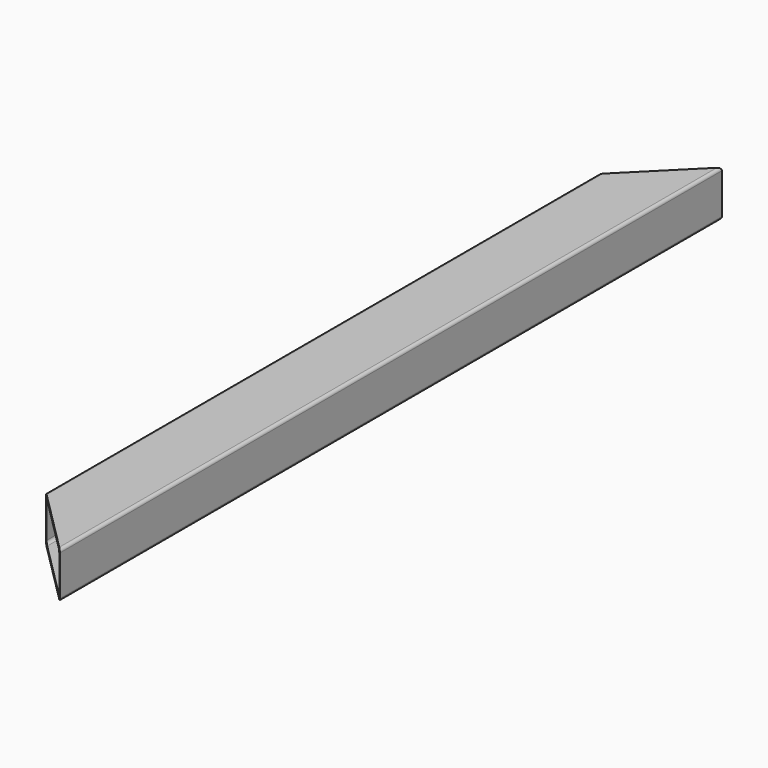
from build123d import *

# Parameters (mm, degrees)
F2_DEPTH = 914.4
F4_DEPTH = 50.801
F6_DEPTH = 50.801
F7_R     = 3.175


# Not quite as in the source:
# - a variable given as a bare number and used for a length is read in inches; the dataset says mm whatever the document's units were


with BuildPart() as f2:
    # F0 (on Front) → F2 (new body)
    with BuildSketch(Plane.XZ):
        Polygon((-38.1, 22.225), (-38.1, -22.225), (-38.1, -25.4), (-34.925, -25.4), (34.925, -25.4), (38.1, -25.4), (38.1, -22.225), (38.1, 22.225), (38.1, 25.4), (34.925, 25.4), (-34.925, 25.4), (-38.1, 25.4), align=None)
        with BuildLine():
            ThreePointArc((31.75, 22.225), (33.9950640303, 21.2950640303), (34.925, 19.05))
            Line((34.925, 19.05), (34.925, -19.05))
            ThreePointArc((34.925, -19.05), (33.9950640303, -21.2950640303), (31.75, -22.225))
            Line((31.75, -22.225), (-31.75, -22.225))
            ThreePointArc((-31.75, -22.225), (-33.9950640303, -21.2950640303), (-34.925, -19.05))
            Line((-34.925, -19.05), (-34.925, 19.05))
            ThreePointArc((-34.925, 19.05), (-33.9950640303, 21.2950640303), (-31.75, 22.225))
            Line((-31.75, 22.225), (31.75, 22.225))
        make_face(mode=Mode.SUBTRACT)
    extrude(amount=F2_DEPTH)

    # F3 (on face) → F4 (cut, through all)
    with BuildSketch(Plane.XY.offset(25.4)):
        Polygon((38.1, 0), (-38.1, 0), (-38.1, -76.2), align=None)
    extrude(amount=-F4_DEPTH, mode=Mode.SUBTRACT)

    # F5 (on face) → F6 (cut, through all)
    with BuildSketch(Plane.XY.offset(25.4)):
        Polygon((-38.1, -914.4), (38.1, -914.4), (-38.1, -838.2), align=None)
    extrude(amount=-F6_DEPTH, mode=Mode.SUBTRACT)

    # F7
    f7_edges = [f2.edges().sort_by_distance(p)[0] for p in [
        (-38.1, -457.2, 25.4),
        (-38.1, -457.2, -25.4),
        (38.1, -457.2, 25.4),
        (38.1, -457.2, -25.4),
    ]]
    fillet(f7_edges, radius=F7_R)


solid = f2.part
